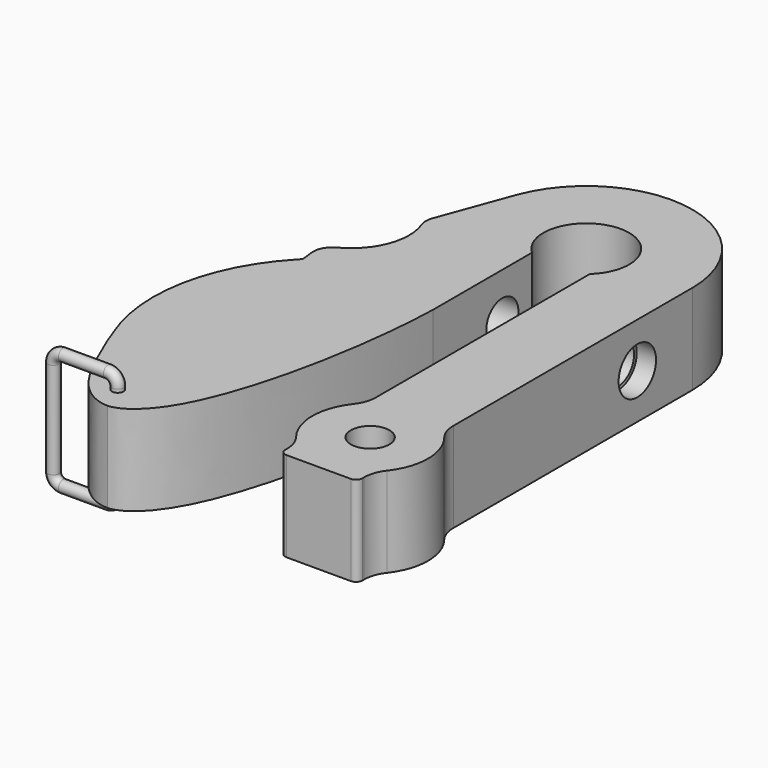
from build123d import *

# Parameters (mm, degrees)
F2_DEPTH  = 14
F3_R      = 3.125
F4_DEPTH  = 49.6420300093
F5_R      = 3
F9_R      = 1
F10_R     = 0.95
F11_DEPTH = 1.5
F12_R     = 0.9
F13_DEPTH = 2.5
F16_R     = 3.64
F17_DEPTH = 3
F19_DEPTH = 14.0010001
F20_R     = 9
F21_DEPTH = 14
F22_R     = 5
F25_DEPTH = 14.0010007
F8_R      = 3
F26_DEPTH = 14.0010012987
F27_R     = 0.95
F28_DEPTH = 2.5
F33_R     = 0.9
F36_R     = 0.9
F37_DEPTH = 1.5


# Not quite as in the source:
# - two fillets or chamfers of one size are made in one step


with BuildPart() as f2:
    # F1 (on Top) → F2 (new body)
    with BuildSketch(Plane.XY):
        with BuildLine():
            Line((-15.4856268226, 5.6960830324), (-20, -6.5768943744))
            ThreePointArc((-20, -6.5768943744), (-19.7757748744, -14.3554235164), (-25.7, -19.4011493494))
            Line((-25.7, -19.4011493494), (-25.2278577536, -23.1385082006))
            add(Edge.make_bspline(
                [(-25.2278577536, -23.1385082006), (-25.1273177564, -23.7020179629), (-25.3713056445, -23.8381959498), (-25.7, -24.2)],
                knots=[0, 0, 0, 0, 1.1617586414, 1.1617586414, 1.1617586414, 1.1617586414], degree=3))
            ThreePointArc((-25.7, -24.2), (-32.6626362635, -37.7529997453), (-31.1790283826, -52.9174652318))
            ThreePointArc((-31.1790283826, -52.9174652318), (-28.6976903426, -62.0182478093), (-28.4015750264, -71.4465879449))
            ThreePointArc((-28.4015750264, -71.4465879449), (-11.4642077603, -64.0498338065), (-4.5, -46.9300735289))
            Line((-4.5, -46.9300735289), (-4.5, -4.9300735289))
            ThreePointArc((-4.5, -4.9300735289), (0, 6.675), (4.5, -4.9300735289))
            Line((4.5, -4.9300735289), (4.5, -65.15))
            Line((4.5, -65.15), (16.5, -65.15))
            Line((16.5, -65.15), (16.5, 0))
            ThreePointArc((16.5, 0), (2.8928495837, 16.2444273918), (-15.4856268226, 5.6960830324))
        make_face()
    extrude(amount=F2_DEPTH)

    # F3 (on face) → F4 (cut, through all)
    with BuildSketch(Plane.YZ.offset(16.5)):
        with Locations((-10.7, 7)):
            Circle(F3_R)
    extrude(amount=-F4_DEPTH, mode=Mode.SUBTRACT)

    # F5
    f5_edges = [f2.edges().sort_by_distance(p)[0] for p in [
        (-20, -6.576894, 7),
        (-25.7, -19.401149, 7),
    ]]
    fillet(f5_edges, radius=F5_R)

    # F9
    f9_edges = [f2.edges().sort_by_distance(p)[0] for p in [
        (4.5, -65.15, 7),
        (16.5, -65.15, 7),
    ]]
    fillet(f9_edges, radius=F9_R)

    # F10 (on Top) → F11 (cut)
    with BuildSketch(Plane.XY):
        with Locations((-21.3149227048, -64.4584521651)):
            Circle(F10_R)
    extrude(amount=F11_DEPTH, mode=Mode.SUBTRACT)

    # F12 (on face) → F13 (cut)
    with BuildSketch(Plane.XY.offset(14)):
        with Locations((-21.3149227048, -64.4584521651)):
            Circle(F12_R)
    extrude(amount=-F13_DEPTH, mode=Mode.SUBTRACT)

    # F16 (on face) → F17 (cut)
    with BuildSketch(Plane.YZ.offset(16.5)):
        with Locations((-10.7, 7)):
            Circle(F16_R)
    extrude(amount=-F17_DEPTH, mode=Mode.SUBTRACT)

    # F18 (on face) → F19 (cut, through all)
    with BuildSketch(Plane.XY.offset(14)):
        with BuildLine():
            ThreePointArc((-28.3963022067, -71.3848695159), (-28.5460846486, -63.1362693547), (-30.3737083693, -55.0912938461))
            Line((-30.3737083693, -55.0912938461), (-30.3737083693, -71.3848695159))
            Line((-30.3737083693, -71.3848695159), (-28.3963022067, -71.3848695159))
        make_face()
        with BuildLine():
            add(Edge.make_bspline(
                [(-30.3737083693, -55.0912938461), (-28.7811456911, -58.7615291796), (-25.6078056235, -67.6579822093), (-18.8855712515, -69.4855479183), (-15.4433224508, -67.3506777059)],
                knots=[0, 0, 0, 0, 0.5347233839, 0.9511026719, 0.9511026719, 0.9511026719, 0.9511026719], degree=3))
            ThreePointArc((-30.3737083693, -55.0912938461), (-28.5460846486, -63.1362693547), (-28.3963022067, -71.3848695159))
            Line((-28.3963022067, -71.3848695159), (-27.1777050831, -71.3848695159))
            ThreePointArc((-27.1777050831, -71.3848695159), (-21.0511507412, -70.1221911319), (-15.4433224508, -67.3506777059))
        make_face()
        with BuildLine():
            add(Edge.make_bspline(
                [(-15.4433224508, -67.3506777059), (-15.0390833975, -67.0999701122), (-14.6279578713, -66.8087869354), (-14.2102387128, -66.474569073)],
                knots=[0.9511026719, 0.9511026719, 0.9511026719, 0.9511026719, 1, 1, 1, 1], degree=3))
            ThreePointArc((-15.4433224508, -67.3506777059), (-21.0511507412, -70.1221911319), (-27.1777050831, -71.3848695159))
            Line((-27.1777050831, -71.3848695159), (-14.2102387128, -71.3848695159))
            Line((-14.2102387128, -71.3848695159), (-14.2102387128, -66.474569073))
        make_face()
        with BuildLine():
            Line((-27.1777050831, -71.3848695159), (-28.3963022067, -71.3848695159))
            ThreePointArc((-28.3963022067, -71.3848695159), (-28.3989267496, -71.4157297442), (-28.4015750264, -71.4465879449))
            ThreePointArc((-28.4015750264, -71.4465879449), (-27.7892545048, -71.4233741447), (-27.1777050831, -71.3848695159))
        make_face()
    extrude(amount=-F19_DEPTH, mode=Mode.SUBTRACT)

    # F20 (on face) → F21 (join)
    with BuildSketch(Plane.XY.offset(14)):
        with Locations((10.4999999818, -55.15)):
            Circle(F20_R)
    extrude(amount=-F21_DEPTH)

    # F22
    f22_edges = [f2.edges().sort_by_distance(p)[0] for p in [
        (16.5, -48.441796, 7),
        (16.5, -61.858204, 7),
        (4.5, -61.858204, 7),
        (4.5, -48.441796, 7),
    ]]
    fillet(f22_edges, radius=F22_R)

    # F24 (on face) → F25 (cut, through all)
    with BuildSketch(Plane.XY.offset(14)):
        with BuildLine():
            add(Edge.make_bspline(
                [(-19.5753466443, -68.5996938374), (-17.4562091898, -68.4435449264), (-9.6242033598, -62.0490559295), (-4.8687699722, -36.9201331283), (-4.5, -24.2009996242)],
                knots=[0.0015878016, 0.0015878016, 0.0015878016, 0.0015878016, 0.3305254663, 1, 1, 1, 1], degree=3))
            Line((-19.5753466443, -68.5996938374), (-19.5753466443, -69.6116682716))
            Line((-19.5753466443, -69.6116682716), (-2.4172839959, -69.6116682716))
            Line((-2.4172839959, -69.6116682716), (-2.4172839959, -24.2009996242))
            Line((-2.4172839959, -24.2009996242), (-4.5, -24.2009996242))
        make_face()
    extrude(amount=-F25_DEPTH, mode=Mode.SUBTRACT)

    # F8 (on face) → F26 (cut, through all)
    with BuildSketch(Plane.XY.offset(14)):
        with Locations((10.5, -55.15)):
            Circle(F8_R)
    extrude(amount=-F26_DEPTH, mode=Mode.SUBTRACT)

    # F27 (on face) → F28 (cut)
    with BuildSketch(Plane.XY):
        with Locations((-21.3149227048, -64.4584521651)):
            Circle(F27_R)
    extrude(amount=F28_DEPTH, mode=Mode.SUBTRACT)

    # F36 (on offset) → F37 (join)
    with BuildSketch(Plane.XY.offset(12.5)):
        with Locations((-21.3149227048, -64.4584521651)):
            Circle(F36_R)
    extrude(amount=-F37_DEPTH)


with BuildPart() as f34:
    # F34: sweep along a path in F31
    with BuildLine(Plane.XZ.offset(64.45845)) as f34_path:
        Line((-21.3149227048, 12.5), (-21.3149227048, 14.5))
        ThreePointArc((-21.3149227048, 14.5), (-21.754262533, 15.5606601718), (-22.8149227048, 16))
        Line((-22.8149227048, 16), (-29.8149227048, 16))
        ThreePointArc((-29.8149227048, 16), (-30.8755828765, 15.5606601718), (-31.3149227048, 14.5))
        Line((-31.3149227048, 14.5), (-31.3149227048, -0.5))
        ThreePointArc((-31.3149227048, -0.5), (-30.8755828765, -1.5606601718), (-29.8149227048, -2))
        Line((-29.8149227048, -2), (-22.8149227048, -2))
        ThreePointArc((-22.8149227048, -2), (-21.754262533, -1.5606601718), (-21.3149227048, -0.5))
        Line((-21.3149227048, -0.5), (-21.3149227048, 1.5))
    # F33 (on offset) → F34 (sweep)
    with BuildSketch(Plane.XY.offset(12.5)):
        with Locations((-21.3149227048, -64.4584521651)):
            Circle(F33_R)
    sweep(path=f34_path.line)


solid = Compound([f2.part, f34.part])
